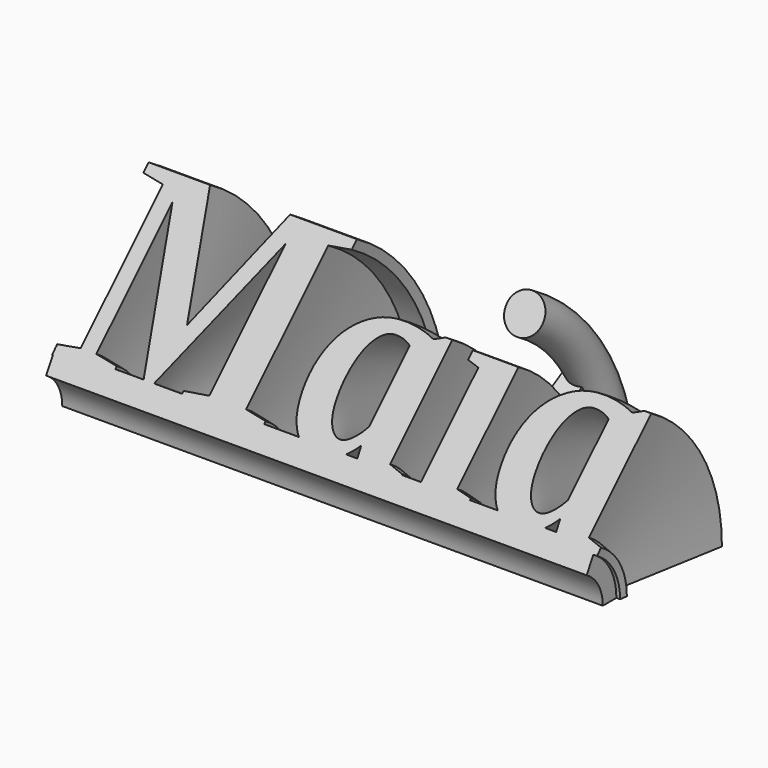
from build123d import *

# Parameters (mm, degrees)
F2_W         = 4.5917695388
F2_H         = 9.3093393371
F4_ANGLE     = 30
F0_TEXT_SIZE = 49.2724033797
F1_W         = 104.1639633477
F1_H         = 4.5288680121
F5_ANGLE     = 60


# Not quite as in the source:
# - Text() gives the source's letters only with a copy of the font that has no kerning and outlines rounded to 1/6400 em; it was checked with that copy


with BuildPart() as f4:
    # F2 (on Top) → F4 (revolve)
    with BuildSketch(Plane.XY):
        with Locations((2.2958847694, 12.0140803047)):
            Rectangle(F2_W, F2_H)
    revolve(axis=Axis((-20.9460128099, -24.5942696929, 0), (1, 0, 0)), revolution_arc=F4_ANGLE)

    # F0 (on Top) + F1 (on Top) → F5 (revolve)
    with BuildSketch(Plane.XY):
        with Locations((-74.9150216579, -13.5237025097)):
            Text('Maia', F0_TEXT_SIZE, font='Tinos', font_style=FontStyle.BOLDITALIC, text_align=(TextAlign.LEFT, TextAlign.BOTTOM))
    with BuildSketch(Plane.XY):
        with Locations((-23.3362521976, -14.5301171578)):
            Rectangle(F1_W, F1_H)
    revolve(axis=Axis((-20.9460128099, -24.5942696929, 0), (1, 0, 0)), revolution_arc=F5_ANGLE)


solid = f4.part
